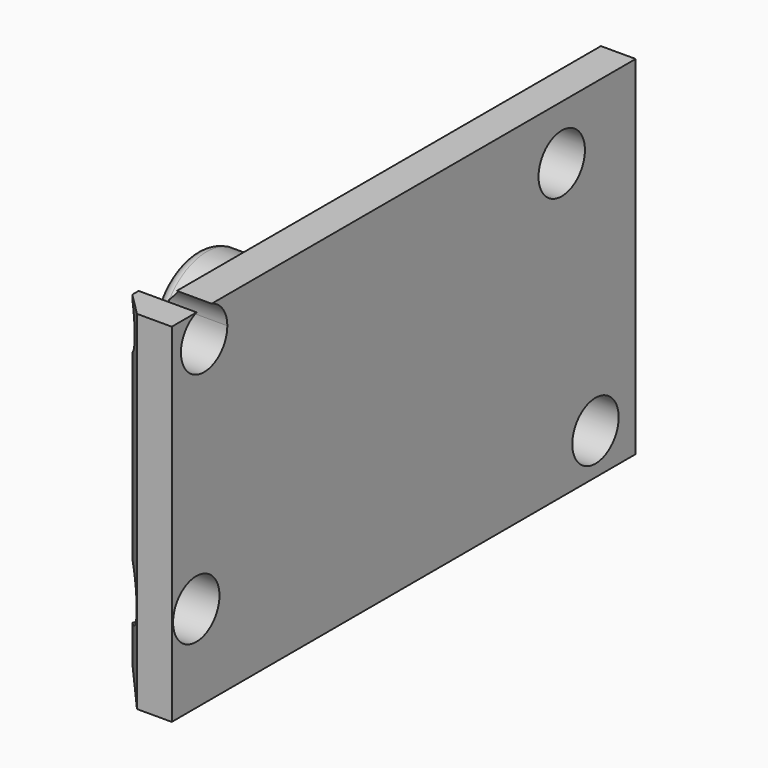
from build123d import *

# Parameters (mm, degrees)
F0_W        = 127
F0_H        = 76.2
F1_DEPTH    = 12.7
F2_R        = 6.35
F3_DEPTH    = 12.701
F4_W        = 7.6199990327
F4_H        = 10.6278949787
F6_R        = 2.54
F7_C1_SIZE  = 5.08
F7_T2_DEPTH = 153.1282991577
F7_T4_DEPTH = 97.2482991577
F7_T6_DEPTH = 92.1682991577


# Not quite as in the source:
# - a fillet or chamfer that OpenCascade refuses, or shapes differently, is made with other operations: its cross-section is extruded or revolved along the edge and cut away or added
# - a feature names something its author has since deleted; it is built from what else it names


with BuildPart() as f1:
    # F0 (on Right) → F1 (new body)
    with BuildSketch(Plane.YZ):
        Rectangle(F0_W, F0_H)
    extrude(amount=F1_DEPTH)

    # F2 (on face) → F3 (cut, through all)
    with BuildSketch(Plane.YZ.offset(12.7)):
        with BuildLine():
            ThreePointArc((-56.6875480297, 38.1), (-58.333550533, 26.9256825374), (-48.2882989585, 32.089752231))
            ThreePointArc((-48.2882989585, 32.089752231), (-49.4742292648, 35.7850038056), (-52.5890498873, 38.1))
            Line((-52.5890498873, 38.1), (-56.6875480297, 38.1))
        make_face()
        with Locations((-56.7933163234, -19.05)):
            Circle(F2_R)
        with Locations((52.4994003593, -29.1107435445)):
            Circle(F2_R)
        with Locations((43.2542454979, 26.190802066)):
            Circle(F2_R)
    extrude(amount=-F3_DEPTH, mode=Mode.SUBTRACT)

    # F4 (on Top) → F5 (revolve)
    with BuildSketch(Plane.XY):
        Polygon((-20.3199990327, -10.6278949787), (-20.3199990327, 0), (-33.0199990327, 0), (-33.0199990327, -12.7), (-20.3199990327, -12.7), align=None)
        with Locations((-16.5099995164, -5.3139474893)):
            Rectangle(F4_W, F4_H)
        Polygon((0, 0), (-12.7, 0), (-12.7, -10.6278949787), (-12.7, -12.7), (0, -12.7), align=None)
    revolve(axis=Axis((-26.6699990327, 0, 0), (1, 0, 0)))

    # F6
    f6_edges = [f1.edges().sort_by_distance(p)[0] for p in [
        (-33.019999, 12.7, 0),
        (0, 12.7, 0),
    ]]
    fillet(f6_edges, radius=F6_R)

    # F7: chamfer of 5.08 on 4 edges, made by hand

    # F7_c1
    f7_c1_edges = [f1.edges().sort_by_distance(p)[0] for p in [
        (0, 5.4554750563, 38.1),
    ]]
    chamfer(f7_c1_edges, length=F7_C1_SIZE)

    # F7_s3 → F7_t2 (cut)
    with BuildSketch(Plane.XZ.offset(-76.5641495789)):
        with BuildLine():
            Line((-0.1436840979, -32.8763159021), (5.2236840979, -38.2436840979))
            Line((5.2236840979, -38.2436840979), (5.2236840979, -38.3452840979))
            ThreePointArc((5.2236840979, -38.3452840979), (2.611842049, -38.2016), (0, -38.2016))
            Line((0, -38.2016), (-0.1016, -38.1))
            ThreePointArc((-0.1016, -38.1), (-0.1016, -35.488157951), (-0.2452840979, -32.8763159021))
            Line((-0.2452840979, -32.8763159021), (-0.1436840979, -32.8763159021))
        make_face()
    extrude(amount=F7_T2_DEPTH, mode=Mode.SUBTRACT)

    # F7_s5 → F7_t4 (cut)
    with BuildSketch(Plane.XY.offset(-46.0841495789)):
        with BuildLine():
            Line((-0.1436840979, -58.2763159021), (5.2236840979, -63.6436840979))
            Line((5.2236840979, -63.6436840979), (5.2236840979, -63.7452840979))
            ThreePointArc((5.2236840979, -63.7452840979), (2.611842049, -63.6016), (0, -63.6016))
            Line((0, -63.6016), (-0.1016, -63.5))
            ThreePointArc((-0.1016, -63.5), (-0.1016, -60.888157951), (-0.2452840979, -58.2763159021))
            Line((-0.2452840979, -58.2763159021), (-0.1436840979, -58.2763159021))
        make_face()
    extrude(amount=F7_T4_DEPTH, mode=Mode.SUBTRACT)

    # F7_s7 → F7_t6 (cut)
    with BuildSketch(Plane.XY.offset(-46.0841495789)):
        with BuildLine():
            Line((-0.1436840979, 58.2763159021), (5.2236840979, 63.6436840979))
            Line((5.2236840979, 63.6436840979), (5.2236840979, 63.7452840979))
            ThreePointArc((5.2236840979, 63.7452840979), (2.611842049, 63.6016), (0, 63.6016))
            Line((0, 63.6016), (-0.1016, 63.5))
            ThreePointArc((-0.1016, 63.5), (-0.1016, 60.888157951), (-0.2452840979, 58.2763159021))
            Line((-0.2452840979, 58.2763159021), (-0.1436840979, 58.2763159021))
        make_face()
    extrude(amount=F7_T6_DEPTH, mode=Mode.SUBTRACT)


solid = f1.part
